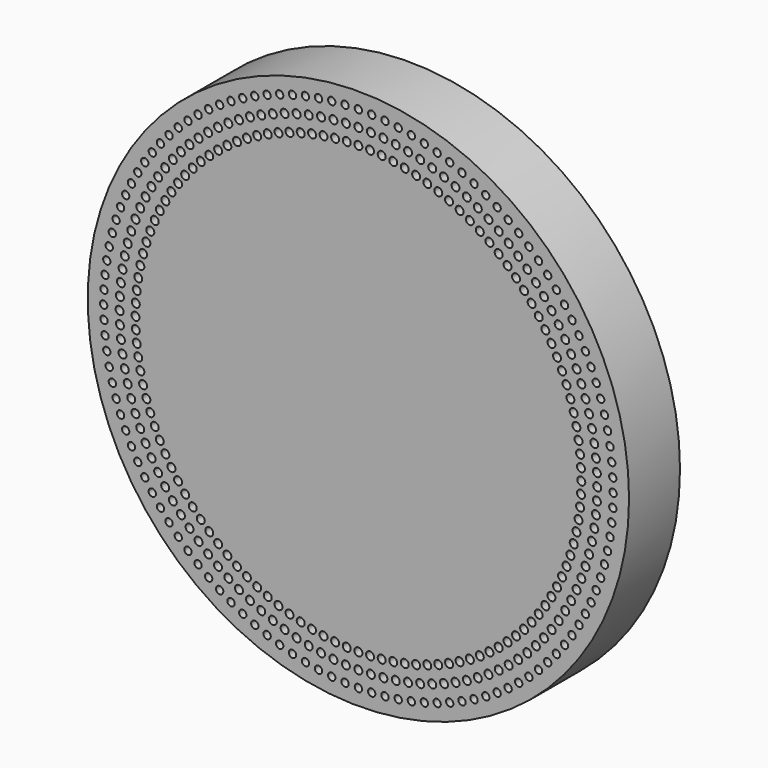
from build123d import *

# Parameters (mm, degrees)
F0_R            = 85
F1_DEPTH        = 20
F2_R            = 1.25
F2_R_2          = 1.2500016794
F2_R_3          = 1.1498638077
F3_DEPTH        = 25
F3_COPIES_COUNT = 120


# Not quite as in the source:
# - a pattern or mirror of a feature is missing from the dataset's text; its kind, count and spacing are read off the source's solid


with BuildPart() as f1:
    # F0 (on Front) → F1 (new body)
    with BuildSketch(Plane.XZ):
        Circle(F0_R)
    extrude(amount=F1_DEPTH)

    # F2 (on face) → F3 (cut)
    with BuildSketch(Plane.XZ.offset(20)):
        with Locations((0, 75)):
            Circle(F2_R)
        with Locations((0, 70)):
            Circle(F2_R_2)
        with Locations((0, 80)):
            Circle(F2_R_3)
    f3 = extrude(amount=-F3_DEPTH, mode=Mode.SUBTRACT)

    # F3_copies: F3 ×120 about axis
    f3_copies_axis = Axis((0, 0, 0), (0, 1, 0))
    for i in range(1, F3_COPIES_COUNT):
        add(f3.rotate(f3_copies_axis, i * 360 / F3_COPIES_COUNT), mode=Mode.SUBTRACT)


solid = f1.part
